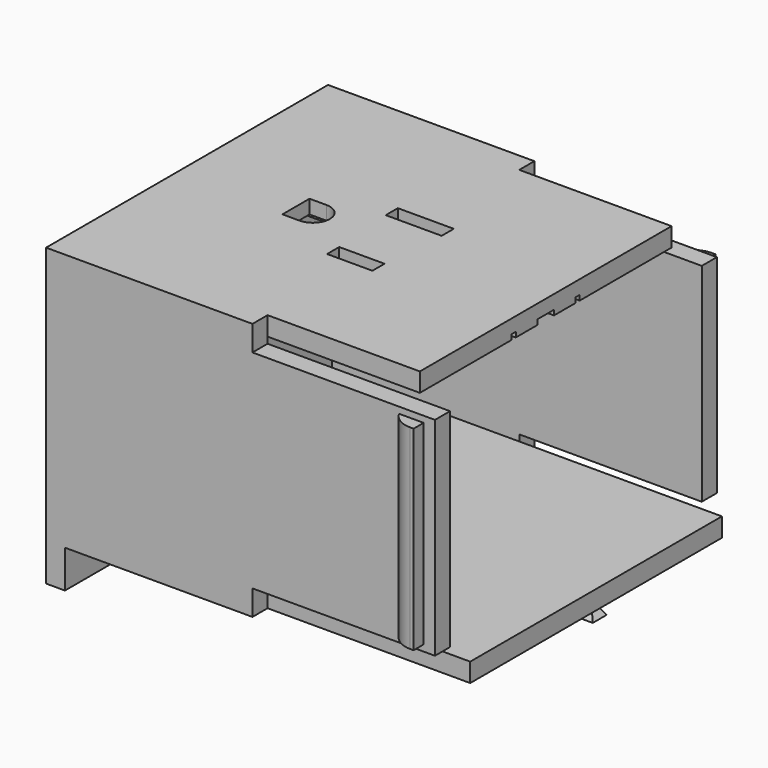
from build123d import *

# Parameters (mm, degrees)
F0_W        = 65
F0_H        = 56
F1_DEPTH    = 41
F2_T        = -3
F3_W        = 5.12
F3_H        = 12.5
F4_DEPTH    = 4.318
F5_W        = 3.9
F5_H        = 31
F6_DEPTH    = 2
F7_W        = 3.9
F7_H        = 31
F8_DEPTH    = 2
F9_T1_DEPTH = 47.7630546142
F11_DEPTH   = 66.294
F12_W       = 8
F12_H       = 50
F13_DEPTH   = 14.732
F14_W       = 8.89
F14_H       = 2.41
F14_W_2     = 7.2
F15_DEPTH   = 25
F16_W       = 7.2
F16_H       = 2.41
F17_DEPTH   = 0.8
F18_W       = 32.2036024
F18_H       = 3
F19_DEPTH   = 25
F20_W       = 32.2036024
F20_H       = 3
F21_DEPTH   = 3.5
F22_W       = 65
F22_H       = 1.6
F23_DEPTH   = 1
F23_TAPER   = -30
F25_DEPTH   = 0.8
F26_W       = 8.89
F26_H       = 2.41
F27_DEPTH   = 0.8
F28_W       = 0.5773502692
F28_H       = 2.7547005384
F29_DEPTH   = 25
F30_W       = 3
F30_H       = 27.2
F30_H_2     = 28.8
F31_DEPTH   = 6


# Not quite as in the source:
# - a fillet or chamfer that OpenCascade refuses, or shapes differently, is made with other operations: its cross-section is extruded or revolved along the edge and cut away or added


with BuildPart() as f1:
    # F0 (on Top) → F1 (new body)
    with BuildSketch(Plane.XY):
        with Locations((-1.2741552845, -5.3390697837)):
            Rectangle(F0_W, F0_H)
    extrude(amount=F1_DEPTH)

    # F2
    f2_openings = [f1.faces().sort_by_distance(p)[0] for p in [
        (31.225845, -5.33907, 20.5),
    ]]
    offset(amount=F2_T, openings=f2_openings)

    # F3 (on face) → F4 (cut)
    with BuildSketch(Plane(origin=(-33.7741552845, 0, 0), x_dir=(0, -1, 0), z_dir=(-1, 0, 0))):
        with Locations((-7.7209302163, 19.25)):
            Rectangle(F3_W, F3_H)
        with Locations((11.3990697837, 19.25)):
            Rectangle(F3_W, F3_H)
    extrude(amount=-F4_DEPTH, mode=Mode.SUBTRACT)

    # F5 (on face) → F6 (join)
    with BuildSketch(Plane(origin=(0, 22.6609302163, 0), x_dir=(-1, 0, 0), z_dir=(0, 1, 0))):
        with Locations((-24.2758447155, 20.5)):
            Rectangle(F5_W, F5_H)
    extrude(amount=F6_DEPTH)

    # F7 (on face) → F8 (join)
    with BuildSketch(Plane.XZ.offset(33.3390697837)):
        with Locations((24.2758447155, 20.5)):
            Rectangle(F7_W, F7_H)
    extrude(amount=F8_DEPTH)

    # F9: fillet of radius 3.81 on 2 edges, made by hand

    # F9_s2 → F9_t1 (cut)
    with BuildSketch(Plane.XY.offset(-3.3815273071)):
        with BuildLine():
            ThreePointArc((22.3258447155, 22.6609302163), (23.7265335088, 24.1229479424), (25.6784556384, 24.6609302163))
            Line((25.6784556384, 24.6609302163), (22.3258447155, 24.6609302163))
            Line((22.3258447155, 24.6609302163), (22.3258447155, 22.6609302163))
        make_face()
        with BuildLine():
            ThreePointArc((22.3258447155, -33.3390697837), (23.7265335088, -34.8010875098), (25.6784556384, -35.3390697837))
            Line((25.6784556384, -35.3390697837), (22.3258447155, -35.3390697837))
            Line((22.3258447155, -35.3390697837), (22.3258447155, -33.3390697837))
        make_face()
    extrude(amount=F9_T1_DEPTH, mode=Mode.SUBTRACT)

    # F10 (on face) → F11 (cut)
    with BuildSketch(Plane(origin=(0, 22.6609302163, 0), x_dir=(-1, 0, 0), z_dir=(0, 1, 0))):
        Polygon((0.9777576845, 38), (-31.2258447155, 38), (-31.2258447155, 3), (0.9777576845, 3), (0.9777576845, 4), (-28.0222423155, 4), (-28.0222423155, 37), (0.9777576845, 37), align=None)
    extrude(amount=-F11_DEPTH, mode=Mode.SUBTRACT)

    # F12 (on face) → F13 (cut)
    with BuildSketch(Plane.XY.offset(41)):
        with Locations((27.2258447155, -5.3390697837)):
            Rectangle(F12_W, F12_H)
    extrude(amount=-F13_DEPTH, mode=Mode.SUBTRACT)

    # F14 (on face) → F15 (cut)
    with BuildSketch(Plane.XY.offset(41)):
        with Locations((-1.8741552845, 1.0109302163)):
            Rectangle(F14_W, F14_H)
        with BuildLine():
            ThreePointArc((-13.7741552845, -8.0290697837), (-11.8720380431, -7.2411870251), (-11.0841552845, -5.3390697837))
            ThreePointArc((-11.0841552845, -5.3390697837), (-11.8720380431, -3.4369525423), (-13.7741552845, -2.6490697837))
            ThreePointArc((-13.7741552845, -2.6490697837), (-15.6762725259, -3.4369525423), (-16.4641552845, -5.3390697837))
            ThreePointArc((-16.4641552845, -5.3390697837), (-15.6762725259, -7.2411870251), (-13.7741552845, -8.0290697837))
        make_face()
        with Locations((-1.8741552845, -11.6890697837)):
            Rectangle(F14_W_2, F14_H)
        with BuildLine():
            ThreePointArc((-16.4641552845, -5.3390697837), (-15.6762725259, -3.4369525423), (-13.7741552845, -2.6490697837))
            Line((-13.7741552845, -2.6490697837), (-16.4641552845, -2.6490697837))
            Line((-16.4641552845, -2.6490697837), (-16.4641552845, -5.3390697837))
        make_face()
        with BuildLine():
            Line((-16.4641552845, -8.0290697837), (-13.7741552845, -8.0290697837))
            ThreePointArc((-13.7741552845, -8.0290697837), (-15.6762725259, -7.2411870251), (-16.4641552845, -5.3390697837))
            Line((-16.4641552845, -5.3390697837), (-16.4641552845, -8.0290697837))
        make_face()
    extrude(amount=-F15_DEPTH, mode=Mode.SUBTRACT)

    # F16 (on face) → F17 (cut)
    with BuildSketch(Plane(origin=(0, 0, 38), x_dir=(1, 0, 0), z_dir=(0, 0, -1))):
        Polygon((-30.7741552845, 12.0888292812), (-30.7741552845, 11.2888292812), (-8.9876995774, 11.2888292812), (-5.4741552845, 10.0590887787), (1.7258447155, 10.0590887787), (5.2393890084, 11.2888292812), (23.2258447155, 11.2888292812), (23.2258447155, 12.0888292812), (5.2393890084, 12.0888292812), (1.7258447155, 13.3185697837), (-5.4741552845, 13.3185697837), (-8.9876995774, 12.0888292812), align=None)
        with Locations((-1.8741552845, 11.6890697837)):
            Rectangle(F16_W, F16_H, mode=Mode.SUBTRACT)
    extrude(amount=-F17_DEPTH, mode=Mode.SUBTRACT)

    # F18 (on face) → F19 (cut)
    with BuildSketch(Plane(origin=(0, 0, 38), x_dir=(1, 0, 0), z_dir=(0, 0, -1))):
        with Locations((15.1240435155, -21.1609302163)):
            Rectangle(F18_W, F18_H)
        Polygon((-0.9777576845, 33.3390697837), (-0.9777576845, 30.3390697837), (23.2258447155, 30.3390697837), (31.2258447155, 30.3390697837), (31.2258447155, 33.3390697837), align=None)
    extrude(amount=-F19_DEPTH, mode=Mode.SUBTRACT)

    # F20 (on face) → F21 (cut)
    with BuildSketch(Plane(origin=(0, 0, 0), x_dir=(1, 0, 0), z_dir=(0, 0, -1))):
        with Locations((15.1240435155, -21.1609302163)):
            Rectangle(F20_W, F20_H)
        with Locations((15.1240435155, 31.8390697837)):
            Rectangle(F20_W, F20_H)
    extrude(amount=-F21_DEPTH, mode=Mode.SUBTRACT)

    # F22 (on face) → F23 (join)
    with BuildSketch(Plane(origin=(0, 0, 0), x_dir=(1, 0, 0), z_dir=(0, 0, -1))):
        with Locations((-1.2741552845, 5.3390697837)):
            Rectangle(F22_W, F22_H)
    extrude(amount=F23_DEPTH, taper=F23_TAPER)

    # F24 (on face) → F25 (cut)
    with BuildSketch(Plane(origin=(0, 0, 38), x_dir=(1, 0, 0), z_dir=(0, 0, -1))):
        Polygon((23.2258447155, 3.6890697837), (23.2258447155, 6.9890697837), (-8.1741552845, 6.9890697837), (-8.9247106344, 8.2890697837), (-8.9247106344, 8.7890697837), (-19.4271999345, 8.7890697837), (-19.4271999345, 1.8890697837), (-8.9247106344, 1.8890697837), (-8.9247106344, 2.3890697837), (-8.1741552845, 3.6890697837), align=None)
        with BuildLine():
            Line((-16.4641552845, 8.0290697837), (-13.7741552845, 8.0290697837))
            ThreePointArc((-13.7741552845, 8.0290697837), (-11.0841552845, 5.3390697837), (-13.7741552845, 2.6490697837))
            Line((-13.7741552845, 2.6490697837), (-16.4641552845, 2.6490697837))
            Line((-16.4641552845, 2.6490697837), (-16.4641552845, 8.0290697837))
        make_face(mode=Mode.SUBTRACT)
    extrude(amount=-F25_DEPTH, mode=Mode.SUBTRACT)

    # F26 (on face) → F27 (cut)
    with BuildSketch(Plane(origin=(0, 0, 38), x_dir=(1, 0, 0), z_dir=(0, 0, -1))):
        Polygon((-30.7741552845, -0.6106897138), (-30.7741552845, -1.4106897138), (-9.8326995774, -1.4106897138), (-6.3191552845, -2.6404302163), (2.5708447155, -2.6404302163), (6.0843890084, -1.4106897138), (23.2258447155, -1.4106897138), (23.2258447155, -0.6106897138), (6.0843890084, -0.6106897138), (2.5708447155, 0.6190507887), (-6.3191552845, 0.6190507887), (-9.8326995774, -0.6106897138), align=None)
        with Locations((-1.8741552845, -1.0109302163)):
            Rectangle(F26_W, F26_H, mode=Mode.SUBTRACT)
    extrude(amount=-F27_DEPTH, mode=Mode.SUBTRACT)

    # F28 (on face) → F29 (cut)
    with BuildSketch(Plane(origin=(0, 0, -1), x_dir=(1, 0, 0), z_dir=(0, 0, -1))):
        with Locations((-34.0628304191, 5.3390697837)):
            Rectangle(F28_W, F28_H)
    extrude(amount=-F29_DEPTH, mode=Mode.SUBTRACT)

    # F30 (on face) → F31 (join)
    with BuildSketch(Plane(origin=(0, 0, 0), x_dir=(1, 0, 0), z_dir=(0, 0, -1))):
        with Locations((-32.2741552845, 19.7390697837)):
            Rectangle(F30_W, F30_H)
        with Locations((-32.2741552845, -8.2609302163)):
            Rectangle(F30_W, F30_H_2)
    extrude(amount=F31_DEPTH)


solid = f1.part
